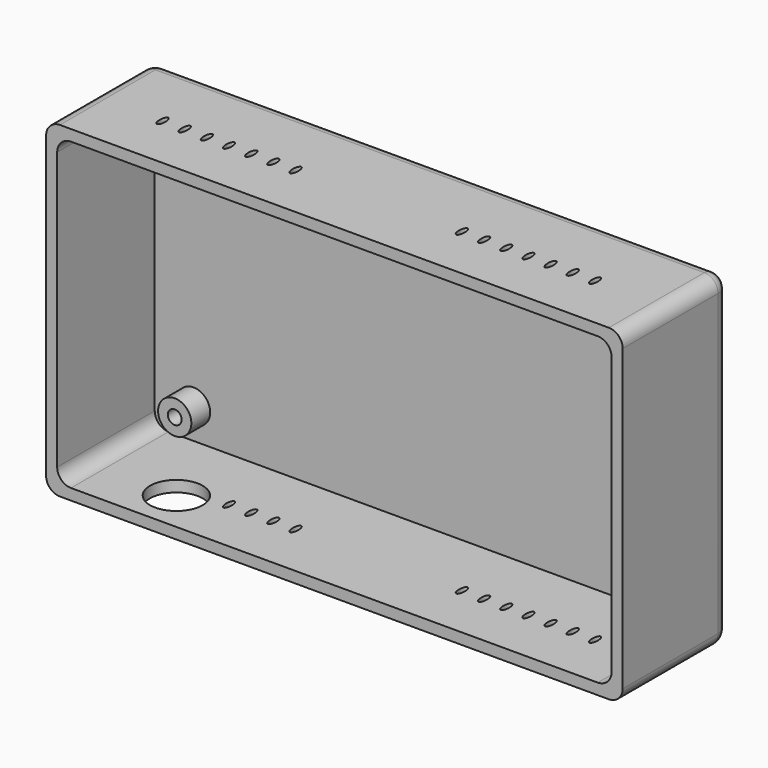
from build123d import *

# Parameters (mm, degrees)
F0_W           = 104
F0_H           = 59
F0_W_2         = 100
F0_H_2         = 55
F2_DEPTH       = 24
F1_W           = 100
F1_H           = 55
F1_R           = 3
F1_R_2         = 1.25
F3_DEPTH       = 2
F4_R           = 2.5
F5_T1_DEPTH    = 27.75
F5_S5_W        = 2.5
F5_S5_H        = 2.5
F5_T6_DEPTH    = 2.5
F5_S11_W       = 2.5
F5_S11_H       = 2.5
F5_T12_DEPTH   = 2.5
F5_S17_W       = 2.5
F5_S17_H       = 2.5
F5_T18_DEPTH   = 2.5
F5_S23_W       = 2.5
F5_S23_H       = 2.5
F5_T24_DEPTH   = 2.5
F6_R           = 2.5
F7_DEPTH       = 6.25
F9_DEPTH       = 59.001
F11_DEPTH      = 25
F11_DEPTH_BACK = 10
F10_R          = 4.75
F12_DEPTH      = 10


# Not quite as in the source:
# - a fillet or chamfer that OpenCascade refuses, or shapes differently, is made with other operations: its cross-section is extruded or revolved along the edge and cut away or added


with BuildPart() as f2:
    # F0 (on Front) → F2 (new body)
    with BuildSketch(Plane.XZ):
        Rectangle(F0_W, F0_H)
        Rectangle(F0_W_2, F0_H_2, mode=Mode.SUBTRACT)
    extrude(amount=F2_DEPTH)

    # F0 (on Front) + F1 (on face) → F3 (join)
    with BuildSketch(Plane.XZ):
        Rectangle(F0_W_2, F0_H_2)
    with BuildSketch(Plane.XZ):
        Rectangle(F1_W, F1_H)
        with Locations((-43, -22)):
            Circle(F1_R, mode=Mode.SUBTRACT)
        with Locations((43, -22)):
            Circle(F1_R, mode=Mode.SUBTRACT)
        with Locations((-43, 22)):
            Circle(F1_R, mode=Mode.SUBTRACT)
        with Locations((43, 22)):
            Circle(F1_R, mode=Mode.SUBTRACT)
        with Locations((43, 22)):
            Circle(F1_R)
        with Locations((43, 22)):
            Circle(F1_R_2, mode=Mode.SUBTRACT)
    extrude(amount=F3_DEPTH)

    # F4
    f4_edges = [f2.edges().sort_by_distance(p)[0] for p in [
        (0, 0, -29.5),
        (0, 0, 29.5),
        (-52, 0, 0),
        (52, 0, 0),
    ]]
    fillet(f4_edges, radius=F4_R)

    # F5: fillet of radius 2.5 on 4 edges, made by hand

    # F5_s2 → F5_t1 (cut)
    with BuildSketch(Plane.XZ.offset(2.5)):
        with BuildLine():
            ThreePointArc((-49.5, 29.5), (-51.267766953, 28.767766953), (-52, 27))
            Line((-52, 27), (-52, 29.5))
            Line((-52, 29.5), (-49.5, 29.5))
        make_face()
        with BuildLine():
            ThreePointArc((49.5, 29.5), (51.267766953, 28.767766953), (52, 27))
            Line((52, 27), (52, 29.5))
            Line((52, 29.5), (49.5, 29.5))
        make_face()
        with BuildLine():
            ThreePointArc((52, -27), (51.267766953, -28.767766953), (49.5, -29.5))
            Line((49.5, -29.5), (52, -29.5))
            Line((52, -29.5), (52, -27))
        make_face()
        with BuildLine():
            ThreePointArc((-52, -27), (-51.267766953, -28.767766953), (-49.5, -29.5))
            Line((-49.5, -29.5), (-52, -29.5))
            Line((-52, -29.5), (-52, -27))
        make_face()
    extrude(amount=F5_T1_DEPTH, mode=Mode.SUBTRACT)


with BuildPart() as f5_tool4:
    # F5_s5 → F5_t6 (new body)
    with BuildSketch(Plane.YZ.offset(-49.5)):
        with Locations((-1.25, -28.25)):
            Rectangle(F5_S5_W, F5_S5_H)
    extrude(amount=-F5_T6_DEPTH)

    # F5_s7 → F5_t8 (revolve, cut)
    with BuildSketch(Plane(origin=(-49.5, -2.5, -27), x_dir=(0, -0.7071067812, 0.7071067812), z_dir=(0, -0.7071067812, -0.7071067812))):
        with BuildLine():
            ThreePointArc((0, -2.5), (2.5, 0), (0, 2.5))
            Line((0, 2.5), (0, -2.5))
        make_face()
    revolve(axis=Axis((-49.5, -2.5, -27), (-1, 0, 0)), mode=Mode.SUBTRACT)


with BuildPart() as f2_1:
    add(f2.part)

    # F5_t3: cut F5_tool4
    add(f5_tool4.part, mode=Mode.SUBTRACT)


with BuildPart() as f5_tool10:
    # F5_s11 → F5_t12 (new body)
    with BuildSketch(Plane.YZ.offset(49.5)):
        with Locations((-1.25, -28.25)):
            Rectangle(F5_S11_W, F5_S11_H)
    extrude(amount=F5_T12_DEPTH)

    # F5_s13 → F5_t14 (revolve, cut)
    with BuildSketch(Plane(origin=(49.5, -2.5, -27), x_dir=(0, -0.7071067812, 0.7071067812), z_dir=(0, 0.7071067812, 0.7071067812))):
        with BuildLine():
            ThreePointArc((0, -2.5), (2.5, 0), (0, 2.5))
            Line((0, 2.5), (0, -2.5))
        make_face()
    revolve(axis=Axis((49.5, -2.5, -27), (1, 0, 0)), mode=Mode.SUBTRACT)


with BuildPart() as f2_2:
    add(f2_1.part)

    # F5_t9: cut F5_tool10
    add(f5_tool10.part, mode=Mode.SUBTRACT)


with BuildPart() as f5_tool16:
    # F5_s17 → F5_t18 (new body)
    with BuildSketch(Plane.XY.offset(27)):
        with Locations((50.75, -1.25)):
            Rectangle(F5_S17_W, F5_S17_H)
    extrude(amount=F5_T18_DEPTH)

    # F5_s19 → F5_t20 (revolve, cut)
    with BuildSketch(Plane(origin=(49.5, -2.5, 27), x_dir=(-0.7071067812, -0.7071067812, 0), z_dir=(-0.7071067812, 0.7071067812, 0))):
        with BuildLine():
            ThreePointArc((0, -2.5), (2.5, 0), (0, 2.5))
            Line((0, 2.5), (0, -2.5))
        make_face()
    revolve(axis=Axis((49.5, -2.5, 27), (0, 0, 1)), mode=Mode.SUBTRACT)


with BuildPart() as f2_3:
    add(f2_2.part)

    # F5_t15: cut F5_tool16
    add(f5_tool16.part, mode=Mode.SUBTRACT)


with BuildPart() as f5_tool22:
    # F5_s23 → F5_t24 (new body)
    with BuildSketch(Plane.XY.offset(27)):
        with Locations((-50.75, -1.25)):
            Rectangle(F5_S23_W, F5_S23_H)
    extrude(amount=F5_T24_DEPTH)

    # F5_s25 → F5_t26 (revolve, cut)
    with BuildSketch(Plane(origin=(-49.5, -2.5, 27), x_dir=(0.7071067812, -0.7071067812, 0), z_dir=(-0.7071067812, -0.7071067812, 0))):
        with BuildLine():
            ThreePointArc((0, -2.5), (2.5, 0), (0, 2.5))
            Line((0, 2.5), (0, -2.5))
        make_face()
    revolve(axis=Axis((-49.5, -2.5, 27), (0, 0, 1)), mode=Mode.SUBTRACT)


with BuildPart() as f2_4:
    add(f2_3.part)

    # F5_t21: cut F5_tool22
    add(f5_tool22.part, mode=Mode.SUBTRACT)

    # F6
    f6_edges = [f2_4.edges().sort_by_distance(p)[0] for p in [
        (-50, -13, -27.5),
        (-50, -13, 27.5),
        (50, -13, 27.5),
        (50, -13, -27.5),
    ]]
    fillet(f6_edges, radius=F6_R)

    # F1 (on face) → F7 (join)
    with BuildSketch(Plane.XZ):
        with Locations((-43, 22)):
            Circle(F1_R)
        with Locations((-43, 22)):
            Circle(F1_R_2, mode=Mode.SUBTRACT)
        with Locations((-43, -22)):
            Circle(F1_R)
        with Locations((-43, -22)):
            Circle(F1_R_2, mode=Mode.SUBTRACT)
        with Locations((43, -22)):
            Circle(F1_R)
        with Locations((43, -22)):
            Circle(F1_R_2, mode=Mode.SUBTRACT)
        with Locations((43, 22)):
            Circle(F1_R)
        with Locations((43, 22)):
            Circle(F1_R_2, mode=Mode.SUBTRACT)
    extrude(amount=F7_DEPTH)

    # F8 (on face) → F9 (cut, through all)
    with BuildSketch(Plane.XY.offset(29.5)):
        with BuildLine():
            add(Edge.make_bspline(
                [(14.5, -14), (14.5, -16.1650635095), (15.25, -15.0825317547), (16, -14), (15.25, -12.9174682453), (14.5, -11.8349364905), (14.5, -14)],
                knots=[4.7123889804, 4.7123889804, 4.7123889804, 6.8067840828, 6.8067840828, 8.9011791852, 8.9011791852, 10.9955742876, 10.9955742876, 10.9955742876], degree=2, weights=[1, 0.5, 1, 0.5, 1, 0.5, 1]))
        make_face()
        with BuildLine():
            add(Edge.make_bspline(
                [(18.5, -14), (18.5, -16.1650635095), (19.25, -15.0825317547), (20, -14), (19.25, -12.9174682453), (18.5, -11.8349364905), (18.5, -14)],
                knots=[4.7123889804, 4.7123889804, 4.7123889804, 6.8067840828, 6.8067840828, 8.9011791852, 8.9011791852, 10.9955742876, 10.9955742876, 10.9955742876], degree=2, weights=[1, 0.5, 1, 0.5, 1, 0.5, 1]))
        make_face()
        with BuildLine():
            add(Edge.make_bspline(
                [(22.5, -14), (22.5, -16.1650635095), (23.25, -15.0825317547), (24, -14), (23.25, -12.9174682453), (22.5, -11.8349364905), (22.5, -14)],
                knots=[4.7123889804, 4.7123889804, 4.7123889804, 6.8067840828, 6.8067840828, 8.9011791852, 8.9011791852, 10.9955742876, 10.9955742876, 10.9955742876], degree=2, weights=[1, 0.5, 1, 0.5, 1, 0.5, 1]))
        make_face()
        with BuildLine():
            add(Edge.make_bspline(
                [(26.5, -14), (26.5, -16.1650635095), (27.25, -15.0825317547), (28, -14), (27.25, -12.9174682453), (26.5, -11.8349364905), (26.5, -14)],
                knots=[4.7123889804, 4.7123889804, 4.7123889804, 6.8067840828, 6.8067840828, 8.9011791852, 8.9011791852, 10.9955742876, 10.9955742876, 10.9955742876], degree=2, weights=[1, 0.5, 1, 0.5, 1, 0.5, 1]))
        make_face()
        with BuildLine():
            add(Edge.make_bspline(
                [(30.5, -14), (30.5, -16.1650635095), (31.25, -15.0825317547), (32, -14), (31.25, -12.9174682453), (30.5, -11.8349364905), (30.5, -14)],
                knots=[4.7123889804, 4.7123889804, 4.7123889804, 6.8067840828, 6.8067840828, 8.9011791852, 8.9011791852, 10.9955742876, 10.9955742876, 10.9955742876], degree=2, weights=[1, 0.5, 1, 0.5, 1, 0.5, 1]))
        make_face()
        with BuildLine():
            add(Edge.make_bspline(
                [(34.5, -14), (34.5, -16.1650635095), (35.25, -15.0825317547), (36, -14), (35.25, -12.9174682453), (34.5, -11.8349364905), (34.5, -14)],
                knots=[4.7123889804, 4.7123889804, 4.7123889804, 6.8067840828, 6.8067840828, 8.9011791852, 8.9011791852, 10.9955742876, 10.9955742876, 10.9955742876], degree=2, weights=[1, 0.5, 1, 0.5, 1, 0.5, 1]))
        make_face()
        with BuildLine():
            add(Edge.make_bspline(
                [(38.5, -14), (38.5, -16.1650635095), (39.25, -15.0825317547), (40, -14), (39.25, -12.9174682453), (38.5, -11.8349364905), (38.5, -14)],
                knots=[4.7123889804, 4.7123889804, 4.7123889804, 6.8067840828, 6.8067840828, 8.9011791852, 8.9011791852, 10.9955742876, 10.9955742876, 10.9955742876], degree=2, weights=[1, 0.5, 1, 0.5, 1, 0.5, 1]))
        make_face()
        with BuildLine():
            add(Edge.make_bspline(
                [(-15.5, -14), (-15.5, -16.1650635095), (-14.75, -15.0825317547), (-14, -14), (-14.75, -12.9174682453), (-15.5, -11.8349364905), (-15.5, -14)],
                knots=[4.7123889804, 4.7123889804, 4.7123889804, 6.8067840828, 6.8067840828, 8.9011791852, 8.9011791852, 10.9955742876, 10.9955742876, 10.9955742876], degree=2, weights=[1, 0.5, 1, 0.5, 1, 0.5, 1]))
        make_face()
        with BuildLine():
            add(Edge.make_bspline(
                [(-19.5, -14), (-19.5, -16.1650635095), (-18.75, -15.0825317547), (-18, -14), (-18.75, -12.9174682453), (-19.5, -11.8349364905), (-19.5, -14)],
                knots=[4.7123889804, 4.7123889804, 4.7123889804, 6.8067840828, 6.8067840828, 8.9011791852, 8.9011791852, 10.9955742876, 10.9955742876, 10.9955742876], degree=2, weights=[1, 0.5, 1, 0.5, 1, 0.5, 1]))
        make_face()
        with BuildLine():
            add(Edge.make_bspline(
                [(-23.5, -14), (-23.5, -16.1650635095), (-22.75, -15.0825317547), (-22, -14), (-22.75, -12.9174682453), (-23.5, -11.8349364905), (-23.5, -14)],
                knots=[4.7123889804, 4.7123889804, 4.7123889804, 6.8067840828, 6.8067840828, 8.9011791852, 8.9011791852, 10.9955742876, 10.9955742876, 10.9955742876], degree=2, weights=[1, 0.5, 1, 0.5, 1, 0.5, 1]))
        make_face()
        with BuildLine():
            add(Edge.make_bspline(
                [(-27.5, -14), (-27.5, -16.1650635095), (-26.75, -15.0825317547), (-26, -14), (-26.75, -12.9174682453), (-27.5, -11.8349364905), (-27.5, -14)],
                knots=[4.7123889804, 4.7123889804, 4.7123889804, 6.8067840828, 6.8067840828, 8.9011791852, 8.9011791852, 10.9955742876, 10.9955742876, 10.9955742876], degree=2, weights=[1, 0.5, 1, 0.5, 1, 0.5, 1]))
        make_face()
    extrude(amount=-F9_DEPTH, mode=Mode.SUBTRACT)

    # F8 (on face) → F11 (cut, two sides)
    with BuildSketch(Plane.XY.offset(29.5)) as f11_sk:
        with BuildLine():
            add(Edge.make_bspline(
                [(-31.5, -14), (-31.5, -16.1650635095), (-30.75, -15.0825317547), (-30, -14), (-30.75, -12.9174682453), (-31.5, -11.8349364905), (-31.5, -14)],
                knots=[4.7123889804, 4.7123889804, 4.7123889804, 6.8067840828, 6.8067840828, 8.9011791852, 8.9011791852, 10.9955742876, 10.9955742876, 10.9955742876], degree=2, weights=[1, 0.5, 1, 0.5, 1, 0.5, 1]))
        make_face()
        with BuildLine():
            add(Edge.make_bspline(
                [(-35.5, -14), (-35.5, -16.1650635095), (-34.75, -15.0825317547), (-34, -14), (-34.75, -12.9174682453), (-35.5, -11.8349364905), (-35.5, -14)],
                knots=[4.7123889804, 4.7123889804, 4.7123889804, 6.8067840828, 6.8067840828, 8.9011791852, 8.9011791852, 10.9955742876, 10.9955742876, 10.9955742876], degree=2, weights=[1, 0.5, 1, 0.5, 1, 0.5, 1]))
        make_face()
        with BuildLine():
            add(Edge.make_bspline(
                [(-39.5, -14), (-39.5, -16.1650635095), (-38.75, -15.0825317547), (-38, -14), (-38.75, -12.9174682453), (-39.5, -11.8349364905), (-39.5, -14)],
                knots=[4.7123889804, 4.7123889804, 4.7123889804, 6.8067840828, 6.8067840828, 8.9011791852, 8.9011791852, 10.9955742876, 10.9955742876, 10.9955742876], degree=2, weights=[1, 0.5, 1, 0.5, 1, 0.5, 1]))
        make_face()
    extrude(amount=-F11_DEPTH, mode=Mode.SUBTRACT)
    extrude(f11_sk.sketch, amount=F11_DEPTH_BACK, mode=Mode.SUBTRACT)

    # F10 (on face) → F12 (cut)
    with BuildSketch(Plane(origin=(0, 0, -29.5), x_dir=(1, 0, 0), z_dir=(0, 0, -1))):
        with Locations((-34.5, 16.5)):
            Circle(F10_R)
    extrude(amount=-F12_DEPTH, mode=Mode.SUBTRACT)


solid = f2_4.part
